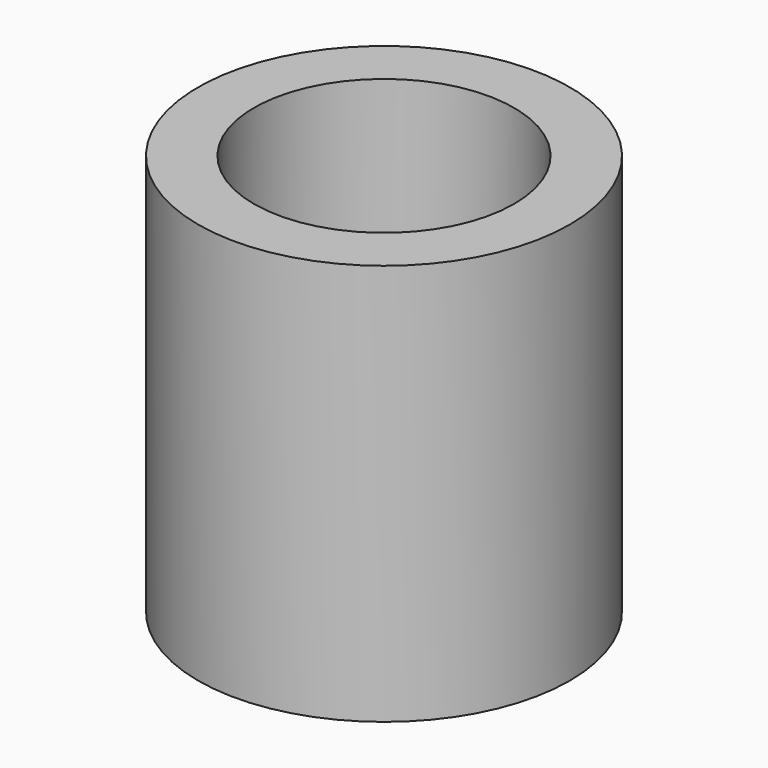
from build123d import *

# Parameters (mm, degrees)
F0_R     = 5
F1_DEPTH = 1
F2_R     = 5
F2_R_2   = 3.5
F3_DEPTH = 9.8


# Not quite as in the source:
# - the program builds the solid bodies; features that only make, move or delete a surface that nothing else refers to are left out


with BuildPart() as f1:
    # F0 (on Top) → F1 (new body)
    with BuildSketch(Plane.XY):
        Circle(F0_R)
    extrude(amount=F1_DEPTH)

    # F2 (on face) → F3 (join)
    with BuildSketch(Plane.XY.offset(1)):
        Circle(F2_R)
        Circle(F2_R_2, mode=Mode.SUBTRACT)
    extrude(amount=F3_DEPTH)


solid = f1.part
